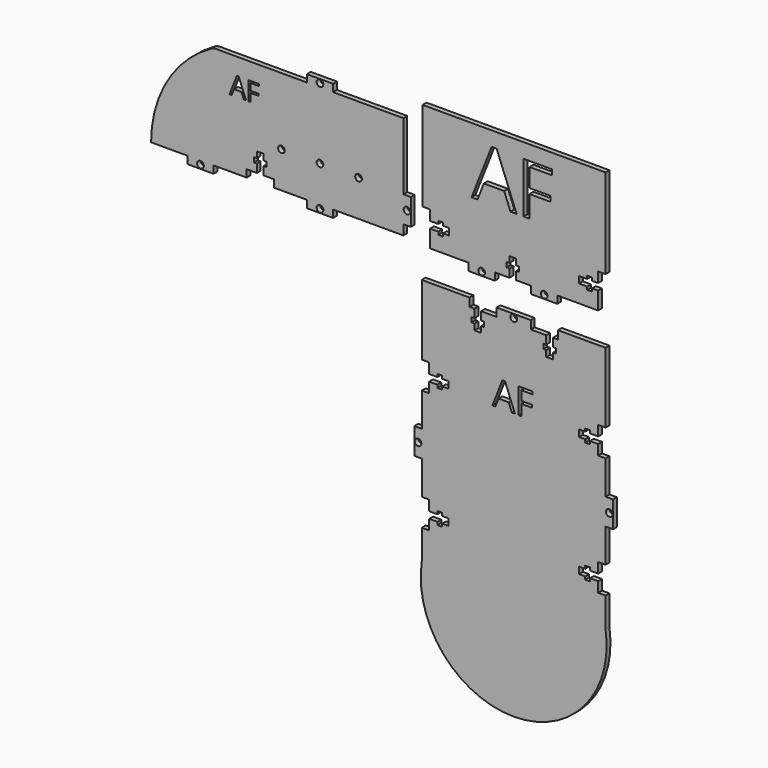
from build123d import *

# Parameters (mm, degrees)
F0_R     = 2.0574
F1_DEPTH = 2.9718
F2_R     = 2.0574
F3_DEPTH = 2.9718
F4_R     = 2.0574
F5_DEPTH = 2.9718
F8_R     = 5.08


# Not quite as in the source:
# - a feature names something its author has since deleted; it is built from what else it names


with BuildPart() as f1:
    # F0 (on Front) → F1 (new body)
    with BuildSketch(Plane.XZ):
        Polygon((-18.5969026979, -10.7412008894), (-18.5969026979, -15.2876914638), (-2.4300471224, -15.2876914638), (-2.4300471224, -10.7412008894), (6.6548, -10.7412008894), (6.6548, -5.6612008894), (4.8768, -5.6612008894), (4.8768, -2.7392187621), (6.6548, -2.7392187621), (6.6548, 0.9935991106), (10.7696, 0.9935991106), (10.7696, -2.7392187621), (12.5476, -2.7392187621), (12.5476, -5.6612008894), (10.7696, -5.6612008894), (10.7696, -10.7412008894), (19.8544471224, -10.7412008894), (19.8544471224, -15.2876914638), (36.0213026979, -15.2876914638), (36.0213026979, -10.7412008894), (58.0559210762, -10.7412008894), (61.0555037856, -10.7412008894), (61.0555037856, -6.2738), (61.0555037856, 0), (57.3217037856, 0), (57.3217037856, -1.778), (54.4007037856, -1.778), (54.4007037856, 0), (49.3207037856, 0), (49.3207037856, 4.1148), (54.4007037856, 4.1148), (54.4007037856, 5.8928), (57.3051609099, 5.8928), (57.3051609099, 4.1148), (61.0555037856, 4.1148), (61.0555037856, 10.3886), (65.6021037856, 10.3886), (65.6021037856, 14.4333135534), (65.6021037856, 65.4587991106), (-46.7687365774, 65.4587991106), (-46.7687365774, 14.3063135534), (-46.7687365774, 10.3886), (-42.2221365774, 10.3886), (-42.2221365774, 4.1148), (-37.1421365774, 4.1148), (-37.1421365774, 5.8928905055), (-34.2144520407, 5.8928905055), (-34.2144520407, 4.1148), (-30.4746365774, 4.1148), (-30.4746365774, 0), (-34.2144520407, 0), (-34.2144520407, -1.7524508294), (-37.1421365774, -1.7524508294), (-37.1421365774, 0), (-42.2221365774, 0), (-42.2221365774, -6.2738), (-42.2221365774, -10.7412008894), (-38.2601322443, -10.7412008894), align=None)
        with Locations((-10.5134749102, -12.9762914638)):
            Circle(F0_R, mode=Mode.SUBTRACT)
        with Locations((27.9378749102, -12.9762914638)):
            Circle(F0_R, mode=Mode.SUBTRACT)
        Polygon((10.9815164304, 25.2240356058), (7.2229586146, 25.2240356058), (3.3345597105, 35.1534619812), (-9.1780209456, 35.1534619812), (-13.0185836593, 25.2240356058), (-16.6951365774, 25.2240356058), (-4.3533994583, 56.5772415317), (-1.2987170152, 56.5772415317), align=None, mode=Mode.SUBTRACT)
        Polygon((18.9018228097, 38.5703327229), (18.9018228097, 25.2240356058), (15.273106082, 25.2240356058), (15.273106082, 56.4474004435), (32.6786456403, 56.4474004435), (32.6786456403, 53.2218744633), (18.9018228097, 53.2218744633), (18.9018228097, 41.7958587031), (31.8449291793, 41.7958587031), (31.8449291793, 38.5703327229), align=None, mode=Mode.SUBTRACT)
    extrude(amount=F1_DEPTH)


with BuildPart() as f3:
    # F2 (on Front) → F3 (new body)
    with BuildSketch(Plane.XZ):
        with BuildLine():
            Line((-79.1750495537, -9.0780625232), (-35.9950495537, -9.0780625232))
            Line((-35.9950495537, -9.0780625232), (-35.9950495537, -2.9524219789))
            Line((-35.9950495537, -2.9524219789), (-31.4484495537, -2.9524219789))
            Line((-31.4484495537, -2.9524219789), (-31.4484495537, 13.2019780211))
            Line((-31.4484495537, 13.2019780211), (-35.9950495537, 13.2019780211))
            Line((-35.9950495537, 13.2019780211), (-35.9950495537, 54.4219374768))
            Line((-35.9950495537, 54.4219374768), (-79.1750495537, 54.4219374768))
            Line((-79.1750495537, 54.4219374768), (-79.1750495537, 58.9685374768))
            Line((-79.1750495537, 58.9685374768), (-95.3294495537, 58.9685374768))
            Line((-95.3294495537, 58.9685374768), (-95.3294495537, 54.4219374768))
            Line((-95.3294495537, 54.4219374768), (-152.6318495537, 54.4219374768))
            ThreePointArc((-152.6318495537, 54.4219374768), (-180.7064304088, 28.0336952904), (-191.0620495537, -9.0780625232))
            Line((-191.0620495537, -9.0780625232), (-168.7862495537, -9.0780625232))
            Line((-168.7862495537, -9.0780625232), (-168.7862495537, -13.6246625232))
            Line((-168.7862495537, -13.6246625232), (-152.6318495537, -13.6246625232))
            Line((-152.6318495537, -13.6246625232), (-152.6318495537, -9.0780625232))
            Line((-152.6318495537, -9.0780625232), (-132.3118495537, -9.0780625232))
            Line((-132.3118495537, -9.0780625232), (-132.3118495537, -4.5314625232))
            Line((-132.3118495537, -4.5314625232), (-126.0380495537, -4.5314625232))
            Line((-126.0380495537, -4.5314625232), (-126.0380495537, 0.5485374768))
            Line((-126.0380495537, 0.5485374768), (-127.8160495537, 0.5485374768))
            Line((-127.8160495537, 0.5485374768), (-127.8160495537, 3.4695374768))
            Line((-127.8160495537, 3.4695374768), (-126.0380495537, 3.4695374768))
            Line((-126.0380495537, 3.4695374768), (-126.0380495537, 7.2160374768))
            Line((-126.0380495537, 7.2160374768), (-121.9232495537, 7.2160374768))
            Line((-121.9232495537, 7.2160374768), (-121.9232495537, 3.4695374768))
            Line((-121.9232495537, 3.4695374768), (-120.1452495537, 3.4695374768))
            Line((-120.1452495537, 3.4695374768), (-120.1452495537, 0.5485374768))
            Line((-120.1452495537, 0.5485374768), (-121.9232495537, 0.5485374768))
            Line((-121.9232495537, 0.5485374768), (-121.9232495537, -4.5314625232))
            Line((-121.9232495537, -4.5314625232), (-115.6494495537, -4.5314625232))
            Line((-115.6494495537, -4.5314625232), (-115.6494495537, -9.0780625232))
            Line((-115.6494495537, -9.0780625232), (-95.3294495537, -9.0780625232))
            Line((-95.3294495537, -9.0780625232), (-95.3294495537, -13.6246625232))
            Line((-95.3294495537, -13.6246625232), (-79.1750495537, -13.6246625232))
            Line((-79.1750495537, -13.6246625232), (-79.1750495537, -9.0780625232))
        make_face()
        with Locations((-160.7090495537, -11.3132625232)):
            Circle(F2_R, mode=Mode.SUBTRACT)
        with Locations((-87.2522495537, -11.3132625232)):
            Circle(F2_R, mode=Mode.SUBTRACT)
        with Locations((-110.9758495537, 13.2019780211)):
            Circle(F2_R, mode=Mode.SUBTRACT)
        with Locations((-87.2522495537, 13.2019780211)):
            Circle(F2_R, mode=Mode.SUBTRACT)
        with Locations((-63.5286495537, 13.2019780211)):
            Circle(F2_R, mode=Mode.SUBTRACT)
        with Locations((-33.7598495537, 5.1247780211)):
            Circle(F2_R, mode=Mode.SUBTRACT)
        Polygon((-132.7194508194, 32.6060913503), (-134.0968957035, 32.6060913503), (-135.5219250472, 36.2450502895), (-140.1075642886, 36.2450502895), (-141.5150625156, 32.6060913503), (-142.8624540567, 32.6060913503), (-138.3394259465, 44.0964861288), (-137.2199389225, 44.0964861288), align=None, mode=Mode.SUBTRACT)
        Polygon((-129.8167987819, 37.4972729114), (-129.8167987819, 32.6060913503), (-131.1466592063, 32.6060913503), (-131.1466592063, 44.0489016692), (-124.7678371704, 44.0489016692), (-124.7678371704, 42.8668035141), (-129.8167987819, 42.8668035141), (-129.8167987819, 38.6793710665), (-125.0733794902, 38.6793710665), (-125.0733794902, 37.4972729114), align=None, mode=Mode.SUBTRACT)
        with Locations((-87.2522495537, 56.6571374768)):
            Circle(F2_R, mode=Mode.SUBTRACT)
    extrude(amount=F3_DEPTH)


with BuildPart() as f5:
    # F4 (on Front) → F5 (new body)
    with BuildSketch(Plane.XZ):
        Polygon((-17.9715745272, -38.5677560119), (-47.3085745272, -38.5677560119), (-47.3085745272, -81.7477560119), (-42.7365745272, -81.7477560119), (-42.7365745272, -88.0215560119), (-37.6600883901, -88.0215560119), (-37.6600883901, -86.2435560119), (-34.7390883901, -86.2435560119), (-34.7529165447, -88.0215560119), (-31.0017745272, -88.0215560119), (-31.0017745272, -92.1363560119), (-34.7390883901, -92.1363560119), (-34.7390883901, -93.9143560119), (-37.6600883901, -93.9143560119), (-37.6600883901, -92.1363560119), (-42.7364388524, -92.1363560119), (-42.7364388524, -98.4101560119), (-47.3085745272, -98.4101560119), (-47.3085745272, -119.1156101778), (-51.8805745272, -119.1156101778), (-51.8805745272, -135.2700101778), (-47.3085745272, -135.2700101778), (-47.3085745272, -155.9710101778), (-42.7365745272, -155.9710101778), (-42.7365745272, -162.2448101778), (-37.6600883901, -162.2448101778), (-37.6600883901, -160.4668101778), (-34.7390883901, -160.4668101778), (-34.7390883901, -162.2448101778), (-31.0017745272, -162.2448101778), (-31.0017745272, -166.3596101778), (-34.7390883901, -166.3596101778), (-34.7390883901, -168.1283563375), (-37.6600883901, -168.1283563375), (-37.6600883901, -166.3596101778), (-42.7365745272, -166.3596101778), (-42.7365745272, -172.6334101778), (-47.3085745272, -172.6334101778), (-47.3085745272, -190.9677560119), (65.6960254728, -190.9677560119), (65.6960254728, -172.6334101778), (61.1240254728, -172.6334101778), (61.1240254728, -166.3596101778), (56.0475393357, -166.3596101778), (56.0475393357, -168.1283563375), (53.1265393357, -168.1283563375), (53.1265393357, -166.3596101778), (49.3892254728, -166.3596101778), (49.3892254728, -162.2448101778), (53.1265393357, -162.2448101778), (53.1265393357, -160.4668101778), (56.0475393357, -160.4668101778), (56.0475393357, -162.2448101778), (61.1240254728, -162.2448101778), (61.1240254728, -155.9710101778), (65.6960254728, -155.9710101778), (65.6960254728, -135.2700101778), (65.801076591, -135.2700101778), (70.2680254728, -135.2700101778), (70.2680254728, -119.1156101778), (65.6960254728, -119.1156101778), (65.6960254728, -98.4101560119), (61.123889798, -98.4101560119), (61.123889798, -92.1363560119), (56.0475393357, -92.1363560119), (56.0475393357, -93.9143560119), (53.1265393357, -93.9143560119), (53.1265393357, -92.1363560119), (49.3892254728, -92.1363560119), (49.3892254728, -88.0215560119), (53.1403674903, -88.0215560119), (53.1265393357, -86.2435560119), (56.0475393357, -86.2435560119), (56.0475393357, -88.0215560119), (61.1240254728, -88.0215560119), (61.1240254728, -81.7477560119), (65.6960254728, -81.7477560119), (65.6960254728, -38.5677560119), (36.3590254728, -38.5677560119), (36.3590254728, -43.6396975759), (33.3237254728, -43.6396975759), (33.3237254728, -48.7196975759), (35.1017254728, -48.7196975759), (35.1017254728, -51.6445748508), (33.3237254728, -51.6445748508), (33.3237254728, -55.3744975759), (29.2089254728, -55.3744975759), (29.2089254728, -51.6445748508), (27.4309254728, -51.6445748508), (27.4309254728, -48.7196975759), (29.2089254728, -48.7196975759), (29.2089254728, -43.6396975759), (19.6966254728, -43.6396975759), (19.6966254728, -38.5677560119), (9.1937254728, -38.5677560119), (-1.3091745272, -38.5677560119), (-1.3091745272, -43.6396975759), (-10.8214745272, -43.6396975759), (-10.8214745272, -48.7196975759), (-9.0434745272, -48.7196975759), (-9.0434745272, -51.6445748508), (-10.8214745272, -51.6445748508), (-10.8214745272, -55.3744975759), (-14.9362745272, -55.3744975759), (-14.9362745272, -51.6445748508), (-16.7142745272, -51.6445748508), (-16.7142745272, -48.7196975759), (-14.9362745272, -48.7196975759), (-14.9362745272, -43.6396975759), (-17.9715745272, -43.6396975759), align=None)
        with Locations((-49.5691745272, -127.1928101778)):
            Circle(F4_R, mode=Mode.SUBTRACT)
        Polygon((9.981662249, -92.4006327987), (8.0983238721, -92.4006327987), (6.1499247149, -87.425195232), (-0.1198799544, -87.425195232), (-2.0443093504, -92.4006327987), (-3.8865567082, -92.4006327987), (2.2976416712, -76.6901664837), (3.8282821339, -76.6901664837), align=None, mode=Mode.SUBTRACT)
        with BuildLine():
            ThreePointArc((11.2511254728, -40.8791560119), (7.7389239812, -42.3339575035), (9.1937254728, -38.8217560119))
            ThreePointArc((9.1937254728, -38.8217560119), (10.6485269644, -39.4243545203), (11.2511254728, -40.8791560119))
        make_face(mode=Mode.SUBTRACT)
        with Locations((67.9566254728, -127.1928101778)):
            Circle(F4_R, mode=Mode.SUBTRACT)
        Polygon((13.9503698469, -85.7130694349), (13.9503698469, -92.4006327987), (12.1320922503, -92.4006327987), (12.1320922503, -76.755227264), (20.8536610612, -76.755227264), (20.8536610612, -78.3714740165), (13.9503698469, -78.3714740165), (13.9503698469, -84.0968226823), (20.4359023666, -84.0968226823), (20.4359023666, -85.7130694349), align=None, mode=Mode.SUBTRACT)
        with BuildLine():
            Line((65.6960254728, -190.9677560119), (-47.3085745272, -190.9677560119))
            ThreePointArc((-47.3085745272, -190.9677560119), (9.1937254728, -256.5068706753), (65.6960254728, -190.9677560119))
        make_face()
    extrude(amount=F5_DEPTH)


with BuildPart() as f3_1:
    # F6: moved
    add(f3.part.moved(Location((-22.606, 0, 0))))

    # F8
    f8_edges = [f3_1.edges().sort_by_distance(p)[0] for p in [
        (-175.23785, -1.4859, 54.421937),
    ]]
    fillet(f8_edges, radius=F8_R)


with BuildPart() as f5_1:
    # F7: moved
    add(f5.part.moved(Location((0, 0, 9.144))))


solid = Compound([f1.part, f3_1.part, f5_1.part])
